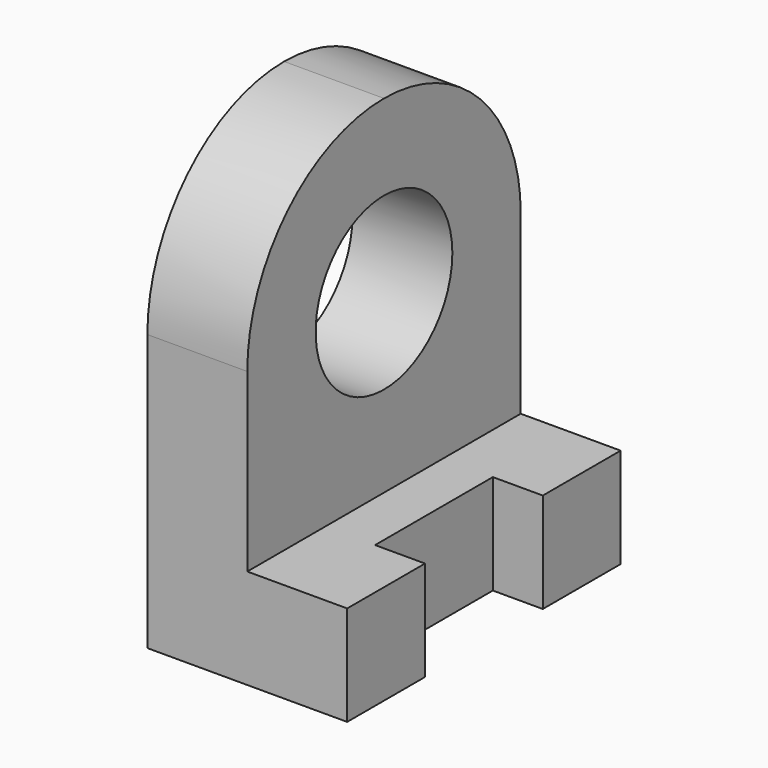
from build123d import *

# Parameters (mm, degrees)
F1_DEPTH = 66.04
F2_R     = 33.02
F3_R     = 33.01999
F4_R     = 16.51
F5_DEPTH = 34.544
F7_DEPTH = 25.4


# Not quite as in the source:
# - a fillet or chamfer is up to 0.001 mm smaller than in the source, because OpenCascade refuses the exact size


with BuildPart() as f1:
    # F0 (on Front) → F1 (new body)
    with BuildSketch(Plane.XZ):
        Polygon((0, 86.36), (0, 0), (38.608, 0), (38.608, 19.304), (19.304, 19.304), (19.304, 86.36), align=None)
    extrude(amount=F1_DEPTH)

    # F2
    f2_edges = [f1.edges().sort_by_distance(p)[0] for p in [
        (9.652, 0, 86.36),
    ]]
    fillet(f2_edges, radius=F2_R)

    # F3 (radius 33.02 in the source; OpenCascade refuses exactly that, so slightly less here)
    f3_edges = [f1.edges().sort_by_distance(p)[0] for p in [
        (9.652, -66.04, 86.36),
    ]]
    fillet(f3_edges, radius=F3_R)

    # F4 (on face) → F5 (cut)
    with BuildSketch(Plane.YZ.offset(19.304)):
        with Locations((-33.02, 53.34)):
            Circle(F4_R)
    extrude(amount=-F5_DEPTH, mode=Mode.SUBTRACT)

    # F6 (on face) → F7 (cut)
    with BuildSketch(Plane.XY.offset(19.304)):
        Polygon((38.608, -47.244), (38.608, -33.02), (38.608, -18.796), (28.956, -18.796), (28.956, -47.244), align=None)
    extrude(amount=-F7_DEPTH, mode=Mode.SUBTRACT)


solid = f1.part
